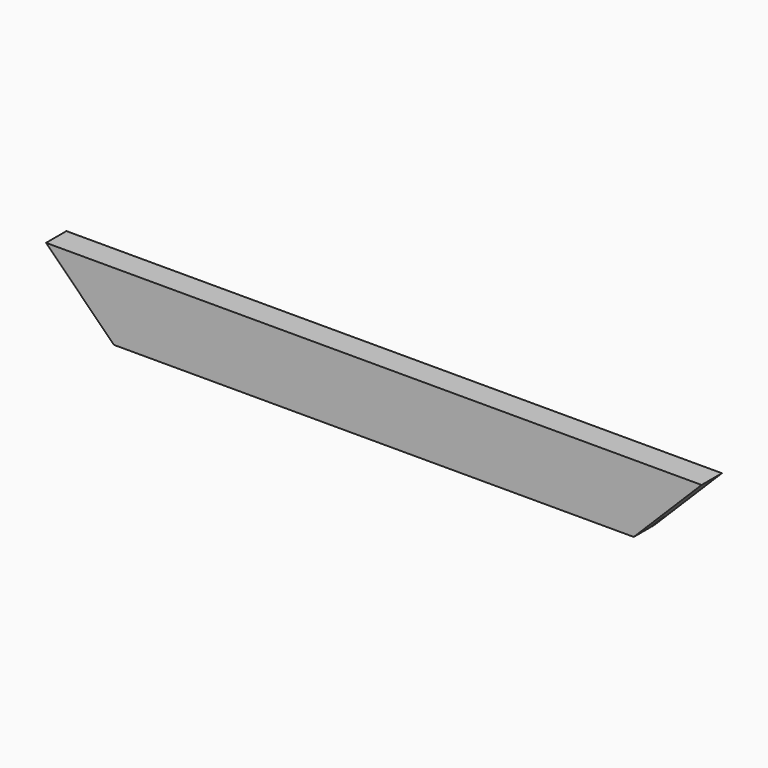
from build123d import *

# Parameters (mm, degrees)
F1_DEPTH = 28.575
F2_W     = 83.9999222453
F2_H     = 3.175
F2_W_2   = 584.2
F2_W_3   = 88.7867628519
F3_DEPTH = 15.875


# Not quite as in the source:
# - a length typed as a fraction of an inch, garbled in the dataset ("3 / 203.2 mm" for 3/8 in), is restored


with BuildPart() as f1:
    # F0 (on Front) → F1 (new body)
    with BuildSketch(Plane.XZ):
        Polygon((-671.1992633168, 21.6867477232), (-594.9992633168, -54.5132522768), (-10.7992633168, -54.5132522768), (65.4007366832, 21.6867477232), align=None)
    extrude(amount=F1_DEPTH)

    # F2 (on face) → F3 (cut)
    with BuildSketch(Plane(origin=(0, 0, -54.5132522768), x_dir=(1, 0, 0), z_dir=(0, 0, -1))):
        with Locations((-636.9992244395, 4.7625)):
            Rectangle(F2_W, F2_H)
        with Locations((-302.8992633168, 4.7625)):
            Rectangle(F2_W_2, F2_H)
        with Locations((33.5941181091, 4.7625)):
            Rectangle(F2_W_3, F2_H)
    extrude(amount=-F3_DEPTH, mode=Mode.SUBTRACT)


solid = f1.part
